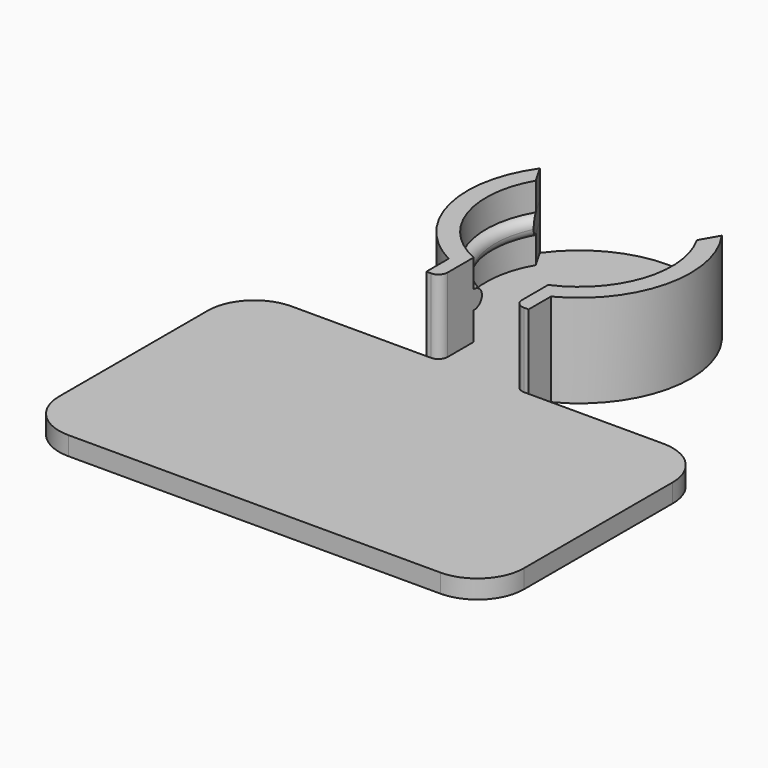
from build123d import *

# Parameters (mm, degrees)
F1_DEPTH  = 2
F3_DEPTH  = 3
F5_DEPTH  = 2
F7_DEPTH  = 3
F8_R      = 0.99999
F9_W      = 20
F9_H      = 14.6653645039
F10_DEPTH = 8
F11_W     = 50
F11_H     = 30
F12_DEPTH = 2
F13_R     = 1
F14_R     = 5


# Not quite as in the source:
# - a fillet or chamfer is up to 0.001 mm smaller than in the source, because OpenCascade refuses the exact size


with BuildPart() as f1:
    # F0 (on Top) → F1 (new body)
    with BuildSketch(Plane.XY):
        with BuildLine():
            ThreePointArc((5.5, 1.5), (0, 24.1653645039), (-5.5, 1.5))
            Line((-5.5, 1.5), (-5.5, -1.5))
            ThreePointArc((-5.5, -1.5), (0, -24.1653645039), (5.5, -1.5))
            Line((5.5, -1.5), (5.5, 1.5))
        make_face()
    extrude(amount=F1_DEPTH)

    # F2 (on face) → F3 (join)
    with BuildSketch(Plane.XY.offset(2)):
        with BuildLine():
            Line((9.7844830762, 19.1125863177), (8.6602540378, 17.1653645039))
            ThreePointArc((8.6602540378, 17.1653645039), (9.4991255677, 9.0402063559), (4, 3.0002131139))
            Line((4, 3.0002131139), (4, -6.2432010007))
            Line((4, -6.2432010007), (9.1651513899, -16.1653645039))
            ThreePointArc((9.1651513899, -16.1653645039), (9.5868378212, -9.3206253964), (5.5, -3.8137179596))
            Line((5.5, -3.8137179596), (5.5, 1.5))
            ThreePointArc((5.5, 1.5), (11.6599594736, 9.3289327537), (9.7844830762, 19.1125863177))
        make_face()
        with BuildLine():
            ThreePointArc((-4, 3.0002131139), (-9.4991255677, 9.0402063559), (-8.6602540378, 17.1653645039))
            Line((-8.6602540378, 17.1653645039), (-9.7844830762, 19.1125863177))
            ThreePointArc((-9.7844830762, 19.1125863177), (-11.6599594736, 9.3289327537), (-5.5, 1.5))
            Line((-5.5, 1.5), (-5.5, -3.8137179596))
            ThreePointArc((-5.5, -3.8137179596), (-9.5868378212, -9.3206253964), (-9.1651513899, -16.1653645039))
            Line((-9.1651513899, -16.1653645039), (-4, -6.2432010007))
            Line((-4, -6.2432010007), (-4, 3.0002131139))
        make_face()
    extrude(amount=F3_DEPTH)

    # F4 (on face) → F5 (join)
    with BuildSketch(Plane.XY.offset(5)):
        with BuildLine():
            Line((-8.0717844057, 16.1461052023), (-9.7844830762, 19.1125863177))
            ThreePointArc((-9.7844830762, 19.1125863177), (-11.6599594736, 9.3289327537), (-5.5, 1.5))
            Line((-5.5, 1.5), (-5.5, -5.0414610795))
            ThreePointArc((-5.5, -5.0414610795), (-8.6043935433, -9.5263473097), (-8.5483759414, -14.980549891))
            Line((-8.5483759414, -14.980549891), (-4, -6.2432010007))
            Line((-4, -6.2432010007), (-4, 4.1031067556))
            ThreePointArc((-4, 4.1031067556), (-8.5258693153, 9.2827350759), (-8.0717844057, 16.1461052023))
        make_face()
        with BuildLine():
            ThreePointArc((5.5, 1.5), (11.6599594736, 9.3289327537), (9.7844830762, 19.1125863177))
            Line((9.7844830762, 19.1125863177), (8.0717844057, 16.1461052023))
            ThreePointArc((8.0717844057, 16.1461052023), (8.5258693153, 9.2827350759), (4, 4.1031067556))
            Line((4, 4.1031067556), (4, -6.2432010007))
            Line((4, -6.2432010007), (8.5483759414, -14.980549891))
            ThreePointArc((8.5483759414, -14.980549891), (8.6043935433, -9.5263473097), (5.5, -5.0414610795))
            Line((5.5, -5.0414610795), (5.5, 1.5))
        make_face()
    extrude(amount=F5_DEPTH)

    # F6 (on face) → F7 (join)
    with BuildSketch(Plane.XY.offset(7)):
        with BuildLine():
            Line((9.7844830762, 19.1125863177), (8.6602540378, 17.1653645039))
            ThreePointArc((8.6602540378, 17.1653645039), (9.4991255677, 9.0402063559), (4, 3.0002131139))
            Line((4, 3.0002131139), (4, -6.2432010007))
            Line((4, -6.2432010007), (9.1651513899, -16.1653645039))
            ThreePointArc((9.1651513899, -16.1653645039), (9.5868378212, -9.3206253964), (5.5, -3.8137179596))
            Line((5.5, -3.8137179596), (5.5, 1.5))
            ThreePointArc((5.5, 1.5), (11.6599594736, 9.3289327537), (9.7844830762, 19.1125863177))
        make_face()
        with BuildLine():
            ThreePointArc((-4, 3.0002131139), (-9.4991255677, 9.0402063559), (-8.6602540378, 17.1653645039))
            Line((-8.6602540378, 17.1653645039), (-9.7844830762, 19.1125863177))
            ThreePointArc((-9.7844830762, 19.1125863177), (-11.6599594736, 9.3289327537), (-5.5, 1.5))
            Line((-5.5, 1.5), (-5.5, -3.8137179596))
            ThreePointArc((-5.5, -3.8137179596), (-9.5868378212, -9.3206253964), (-9.1651513899, -16.1653645039))
            Line((-9.1651513899, -16.1653645039), (-4, -6.2432010007))
            Line((-4, -6.2432010007), (-4, 3.0002131139))
        make_face()
    extrude(amount=F7_DEPTH)

    # F8 (radius 1 in the source; OpenCascade refuses exactly that, so slightly less here)
    f8_edges = [f1.edges().sort_by_distance(p)[0] for p in [
        (8.525869, 9.282735, 7),
        (-8.525869, 9.282735, 7),
        (-8.525869, 9.282735, 5),
        (8.525869, 9.282735, 5),
        (-8.604394, -9.526347, 5),
        (-8.604394, -9.526347, 7),
        (8.604394, -9.526347, 7),
        (8.604394, -9.526347, 5),
    ]]
    fillet(f8_edges, radius=F8_R)

    # F9 (on face) → F10 (cut)
    with BuildSketch(Plane.XY.offset(10)):
        with Locations((0, -8.8326822519)):
            Rectangle(F9_W, F9_H)
    extrude(amount=-F10_DEPTH, mode=Mode.SUBTRACT)

    # F11 (on face) → F12 (join)
    with BuildSketch(Plane.XY.offset(2)):
        with Locations((0, -16.5)):
            Rectangle(F11_W, F11_H)
    extrude(amount=-F12_DEPTH)

    # F13
    f13_edges = [f1.edges().sort_by_distance(p)[0] for p in [
        (-4, -1.5, 6),
        (4, -1.5, 6),
    ]]
    fillet(f13_edges, radius=F13_R)

    # F14
    f14_edges = [f1.edges().sort_by_distance(p)[0] for p in [
        (-25, -1.5, 1),
        (-25, -31.5, 1),
        (25, -31.5, 1),
        (25, -1.5, 1),
    ]]
    fillet(f14_edges, radius=F14_R)


solid = f1.part
